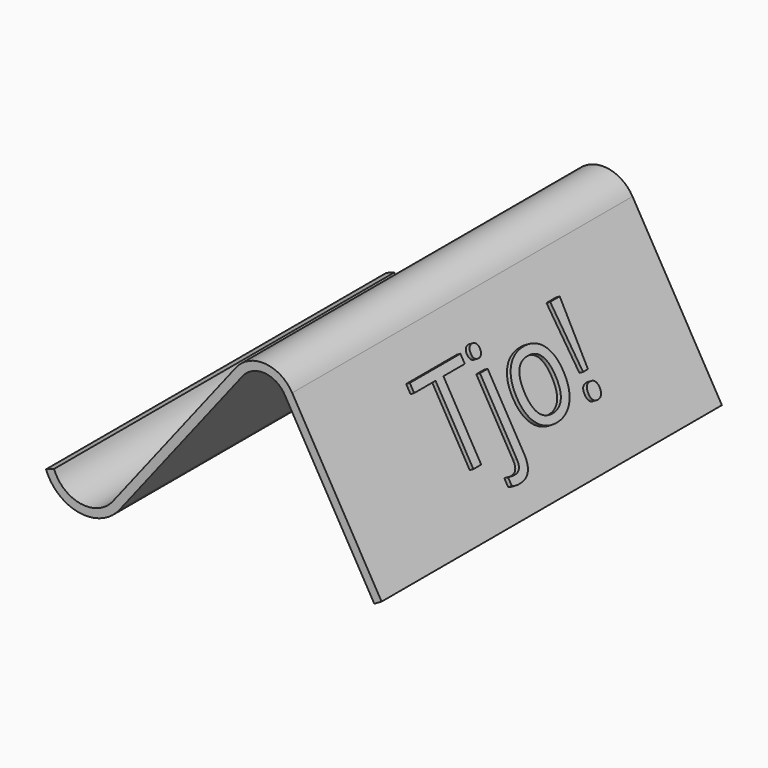
from build123d import *

# Parameters (mm, degrees)
F1_DEPTH     = 100
F2_TEXT_SIZE = 27.7777777778
F3_DEPTH     = 1


# Not quite as in the source:
# - Text() gives the source's letters only with a copy of the font that has no kerning and outlines rounded to 1/6400 em; it was checked with that copy


with BuildPart() as f1:
    # F0 (on Front) → F1 (new body)
    with BuildSketch(Plane.XZ):
        with BuildLine():
            ThreePointArc((-51.6739467822, 2.7423553432), (-43.8404609154, -3.7238580402), (-34.3901541668, 0))
            Line((-34.3901541668, 0), (-5.4729582171, 37.0512587965))
            ThreePointArc((-5.4729582171, 37.0512587965), (-0.3275242067, 39.345298856), (4.4516113795, 36.3623516559))
            Line((4.4516113795, 36.3623516559), (25.4701599035, 0))
            Line((25.4701599035, 0), (27.2017004585, 1.000883263))
            Line((27.2017004585, 1.000883263), (6.1831519345, 37.3632349189))
            ThreePointArc((6.1831519345, 37.3632349189), (-0.1890288471, 41.3404978524), (-7.0496075276, 38.2817777731))
            Line((-7.0496075276, 38.2817777731), (-35.9668034773, 1.2305189766))
            ThreePointArc((-35.9668034773, 1.2305189766), (-43.5270488762, -1.7485674555), (-49.7938375696, 3.4244032511))
            Line((-49.7938375696, 3.4244032511), (-51.6739467822, 2.7423553432))
        make_face()
    extrude(amount=F1_DEPTH)

    # F2 (on face) → F3 (join)
    with BuildSketch(Plane(origin=(20.8229070895, 0, 12.0362755196), x_dir=(0, 1, 0), z_dir=(0.8657702775, 0, 0.5004416315))):
        with Locations((-72.5, 0.2536716227)):
            Text('Tjo!', F2_TEXT_SIZE, font='Open Sans', text_align=(TextAlign.LEFT, TextAlign.BOTTOM))
    extrude(amount=F3_DEPTH)


solid = f1.part
